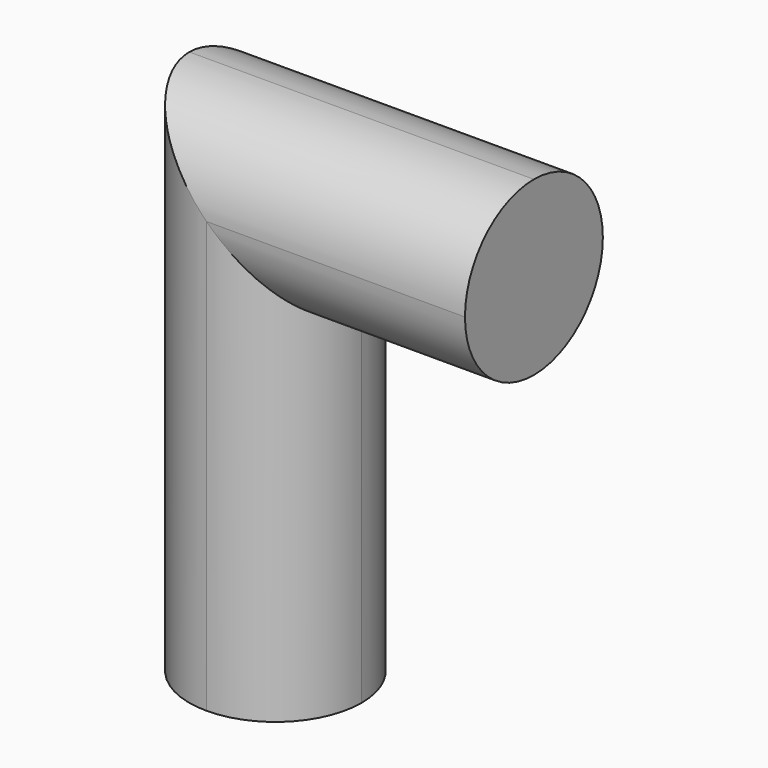
from build123d import *

# Parameters (mm, degrees)
F1_DEPTH = 10
F2_R     = 4.99999


# Not quite as in the source:
# - a fillet or chamfer is up to 0.001 mm smaller than in the source, because OpenCascade refuses the exact size


with BuildPart() as f1:
    # F0 (on Front) → F1 (new body)
    with BuildSketch(Plane.XZ):
        Polygon((0, 30), (0, 0), (10, 0), (10, 20), (20, 20), (20, 30), align=None)
    extrude(amount=F1_DEPTH)

    # F2 (radius 5 in the source; OpenCascade refuses exactly that, so slightly less here)
    f2_edges = [f1.edges().sort_by_distance(p)[0] for p in [
        (10, -10, 30),
        (10, 0, 30),
        (0, -10, 15),
        (10, -10, 10),
        (15, -10, 20),
        (10, 0, 10),
        (15, 0, 20),
        (0, 0, 15),
    ]]
    fillet(f2_edges, radius=F2_R)


solid = f1.part
